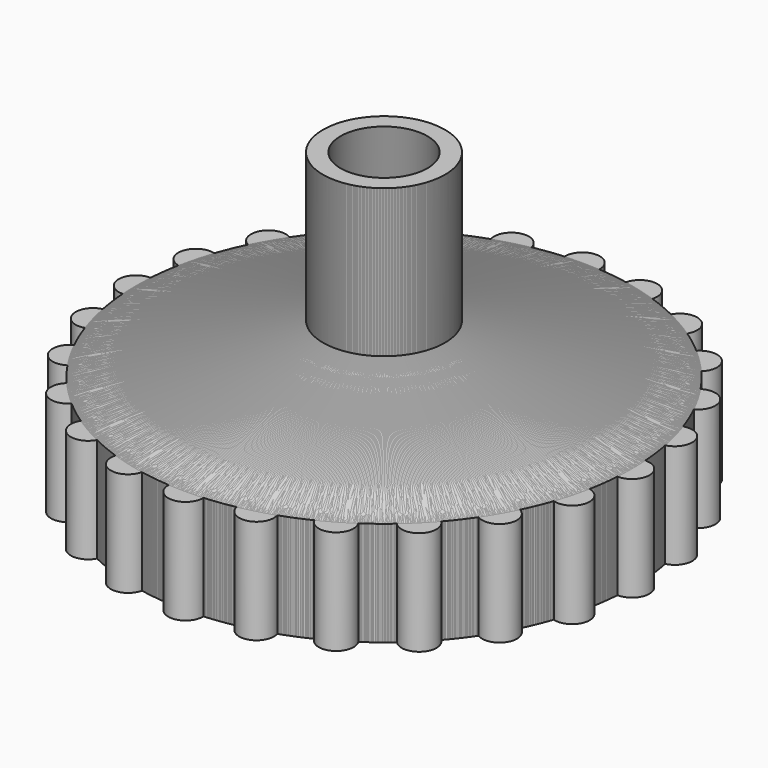
from build123d import *

# Parameters (mm, degrees)
F2_T     = -50.8
F4_DEPTH = 304.8
F5_COUNT = 24


with BuildPart() as f1:
    # F0 (on Front) → F1 (revolve)
    with BuildSketch(Plane.XZ):
        Polygon((0, 0), (0, 882.9270539866), (-177.8, 882.9270539866), (-177.8, 451.1270539866), (-723.9, 304.8), (-723.9, 0), align=None)
    revolve(axis=Axis((0, 0, 56.0227975416), (0, 0, -1)))

    # F2
    f2_openings = [f1.faces().sort_by_distance(p)[0] for p in [
        (0, 0, 882.927054),
        (0, 0, 0),
    ]]
    offset(amount=F2_T, openings=f2_openings, kind=Kind.INTERSECTION)

    # F3 (on face) → F4 (join)
    with BuildSketch(Plane(origin=(0, 0, 0), x_dir=(1, 0, 0), z_dir=(0, 0, -1))):
        with BuildLine():
            ThreePointArc((-50.7687192089, 722.1175438596), (0, 723.9), (50.7687192089, 722.1175438596))
            ThreePointArc((50.7687192089, 722.1175438596), (0, 774.7), (-50.7687192089, 722.1175438596))
        make_face()
    extrude(amount=-F4_DEPTH)


with BuildPart() as f5_1:
    # F5: instance of F1
    add(f1.part.rotate(Axis((0, 0, 304.8), (0, 0, -1)), 1 * 360 / F5_COUNT))


with BuildPart() as f5_2:
    # F5: instance of F1
    add(f1.part.rotate(Axis((0, 0, 304.8), (0, 0, -1)), 2 * 360 / F5_COUNT))


with BuildPart() as f5_3:
    # F5: instance of F1
    add(f1.part.rotate(Axis((0, 0, 304.8), (0, 0, -1)), 3 * 360 / F5_COUNT))


with BuildPart() as f5_4:
    # F5: instance of F1
    add(f1.part.rotate(Axis((0, 0, 304.8), (0, 0, -1)), 4 * 360 / F5_COUNT))


with BuildPart() as f5_5:
    # F5: instance of F1
    add(f1.part.rotate(Axis((0, 0, 304.8), (0, 0, -1)), 5 * 360 / F5_COUNT))


with BuildPart() as f5_6:
    # F5: instance of F1
    add(f1.part.rotate(Axis((0, 0, 304.8), (0, 0, -1)), 6 * 360 / F5_COUNT))


with BuildPart() as f5_7:
    # F5: instance of F1
    add(f1.part.rotate(Axis((0, 0, 304.8), (0, 0, -1)), 7 * 360 / F5_COUNT))


with BuildPart() as f5_8:
    # F5: instance of F1
    add(f1.part.rotate(Axis((0, 0, 304.8), (0, 0, -1)), 8 * 360 / F5_COUNT))


with BuildPart() as f5_9:
    # F5: instance of F1
    add(f1.part.rotate(Axis((0, 0, 304.8), (0, 0, -1)), 9 * 360 / F5_COUNT))


with BuildPart() as f5_10:
    # F5: instance of F1
    add(f1.part.rotate(Axis((0, 0, 304.8), (0, 0, -1)), 10 * 360 / F5_COUNT))


with BuildPart() as f5_11:
    # F5: instance of F1
    add(f1.part.rotate(Axis((0, 0, 304.8), (0, 0, -1)), 11 * 360 / F5_COUNT))


with BuildPart() as f5_12:
    # F5: instance of F1
    add(f1.part.rotate(Axis((0, 0, 304.8), (0, 0, -1)), 12 * 360 / F5_COUNT))


with BuildPart() as f5_13:
    # F5: instance of F1
    add(f1.part.rotate(Axis((0, 0, 304.8), (0, 0, -1)), 13 * 360 / F5_COUNT))


with BuildPart() as f5_14:
    # F5: instance of F1
    add(f1.part.rotate(Axis((0, 0, 304.8), (0, 0, -1)), 14 * 360 / F5_COUNT))


with BuildPart() as f5_15:
    # F5: instance of F1
    add(f1.part.rotate(Axis((0, 0, 304.8), (0, 0, -1)), 15 * 360 / F5_COUNT))


with BuildPart() as f5_16:
    # F5: instance of F1
    add(f1.part.rotate(Axis((0, 0, 304.8), (0, 0, -1)), 16 * 360 / F5_COUNT))


with BuildPart() as f5_17:
    # F5: instance of F1
    add(f1.part.rotate(Axis((0, 0, 304.8), (0, 0, -1)), 17 * 360 / F5_COUNT))


with BuildPart() as f5_18:
    # F5: instance of F1
    add(f1.part.rotate(Axis((0, 0, 304.8), (0, 0, -1)), 18 * 360 / F5_COUNT))


with BuildPart() as f5_19:
    # F5: instance of F1
    add(f1.part.rotate(Axis((0, 0, 304.8), (0, 0, -1)), 19 * 360 / F5_COUNT))


with BuildPart() as f5_20:
    # F5: instance of F1
    add(f1.part.rotate(Axis((0, 0, 304.8), (0, 0, -1)), 20 * 360 / F5_COUNT))


with BuildPart() as f5_21:
    # F5: instance of F1
    add(f1.part.rotate(Axis((0, 0, 304.8), (0, 0, -1)), 21 * 360 / F5_COUNT))


with BuildPart() as f5_22:
    # F5: instance of F1
    add(f1.part.rotate(Axis((0, 0, 304.8), (0, 0, -1)), 22 * 360 / F5_COUNT))


with BuildPart() as f5_23:
    # F5: instance of F1
    add(f1.part.rotate(Axis((0, 0, 304.8), (0, 0, -1)), 23 * 360 / F5_COUNT))


with BuildPart() as f7:
    # F6 (on Front) → F7 (revolve)
    with BuildSketch(Plane.XZ):
        with BuildLine():
            Line((-673.866808414, 215.2970234702), (-673.866808414, 138.8502356224))
            ThreePointArc((-673.866808414, 138.8502356224), (-635.6434144901, 177.0736295463), (-673.866808414, 215.2970234702))
        make_face()
    revolve(axis=Axis((0, 0, 376.1708140373), (0, 0, 1)))


solid = Compound([f1.part, f5_1.part, f5_2.part, f5_3.part, f5_4.part, f5_5.part, f5_6.part, f5_7.part, f5_8.part, f5_9.part, f5_10.part, f5_11.part, f5_12.part, f5_13.part, f5_14.part, f5_15.part, f5_16.part, f5_17.part, f5_18.part, f5_19.part, f5_20.part, f5_21.part, f5_22.part, f5_23.part, f7.part])
